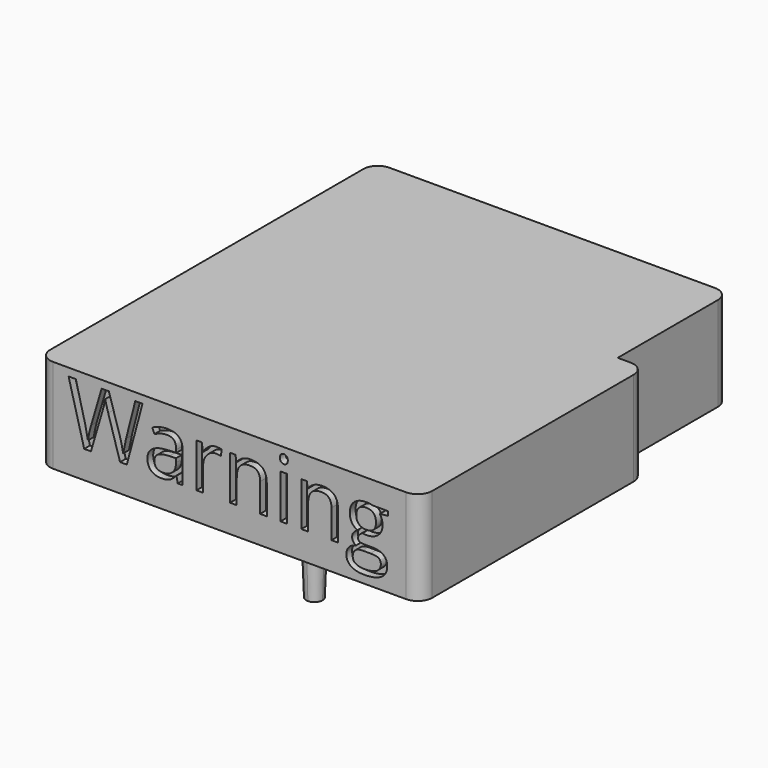
from build123d import *

# Parameters (mm, degrees)
F1_DEPTH     = 10
F2_DEPTH     = 3
F3_DEPTH     = 15
F3_TAPER     = 2
F4_TEXT_SIZE = 11.36543015
F5_DEPTH     = 1


# Not quite as in the source:
# - Text() gives the source's letters only with a copy of the font that has no kerning and outlines rounded to 1/6400 em; it was checked with that copy


with BuildPart() as f1:
    # F0 (on Top) → F1 (new body)
    with BuildSketch(Plane.XY):
        with BuildLine():
            Line((0, 34.5), (0, 0))
            Line((0, 0), (-15, 0))
            ThreePointArc((-15, 0), (-13.833273811, -0.483273811), (-13.35, -1.65))
            ThreePointArc((-13.35, -1.65), (-13.8332738152, -2.8167261931), (-15.0000000118, -3.3))
            Line((-15.0000000118, -3.3), (-1, -3.3))
            ThreePointArc((-1, -3.3), (0.4142135624, -2.7142135624), (1, -1.3))
            Line((1, -1.3), (1, 33.5))
            ThreePointArc((1, 33.5), (0.4142135624, 34.9142135624), (-1, 35.5))
            Line((-1, 35.5), (-2.81, 35.5))
            Line((-2.81, 35.5), (-2.81, 52.8))
            ThreePointArc((-2.81, 52.8), (-3.3957864376, 54.2142135624), (-4.81, 54.8))
            Line((-4.81, 54.8), (-16.51, 54.8))
            ThreePointArc((-16.51, 54.8), (-15.343273811, 54.316726189), (-14.86, 53.15))
            ThreePointArc((-14.86, 53.15), (-15.343273811, 51.983273811), (-16.51, 51.5))
            Line((-16.51, 51.5), (-3.81, 51.5))
            Line((-3.81, 51.5), (-3.81, 34.5))
            Line((-3.81, 34.5), (0, 34.5))
        make_face()
        with BuildLine():
            ThreePointArc((-15.0000000118, -3.3), (-16.65, -1.6499999941), (-15, 0))
            Line((-15, 0), (-50.8, 0))
            Line((-50.8, 0), (-50.8, 51.5))
            Line((-50.8, 51.5), (-16.51, 51.5))
            ThreePointArc((-16.51, 51.5), (-18.16, 53.15), (-16.51, 54.8))
            Line((-16.51, 54.8), (-49.8, 54.8))
            ThreePointArc((-49.8, 54.8), (-51.2142135624, 54.2142135624), (-51.8, 52.8))
            Line((-51.8, 52.8), (-51.8, -1.3))
            ThreePointArc((-51.8, -1.3), (-51.2142135624, -2.7142135624), (-49.8, -3.3))
            Line((-49.8, -3.3), (-15.0000000118, -3.3))
        make_face()
        with BuildLine():
            ThreePointArc((-16.51, 54.8), (-18.16, 53.15), (-16.51, 51.5))
            ThreePointArc((-16.51, 51.5), (-15.343273811, 51.983273811), (-14.86, 53.15))
            ThreePointArc((-14.86, 53.15), (-15.343273811, 54.316726189), (-16.51, 54.8))
        make_face()
        with BuildLine():
            ThreePointArc((-13.35, -1.65), (-13.833273811, -0.483273811), (-15, 0))
            ThreePointArc((-15, 0), (-16.65, -1.6499999941), (-15.0000000118, -3.3))
            ThreePointArc((-15.0000000118, -3.3), (-13.8332738152, -2.8167261931), (-13.35, -1.65))
        make_face()
    extrude(amount=-F1_DEPTH)

    # F0 (on Top) → F2 (join)
    with BuildSketch(Plane.XY):
        with BuildLine():
            Line((0, 34.5), (0, 0))
            Line((0, 0), (-15, 0))
            ThreePointArc((-15, 0), (-13.833273811, -0.483273811), (-13.35, -1.65))
            ThreePointArc((-13.35, -1.65), (-13.8332738152, -2.8167261931), (-15.0000000118, -3.3))
            Line((-15.0000000118, -3.3), (-1, -3.3))
            ThreePointArc((-1, -3.3), (0.4142135624, -2.7142135624), (1, -1.3))
            Line((1, -1.3), (1, 33.5))
            ThreePointArc((1, 33.5), (0.4142135624, 34.9142135624), (-1, 35.5))
            Line((-1, 35.5), (-2.81, 35.5))
            Line((-2.81, 35.5), (-2.81, 52.8))
            ThreePointArc((-2.81, 52.8), (-3.3957864376, 54.2142135624), (-4.81, 54.8))
            Line((-4.81, 54.8), (-16.51, 54.8))
            ThreePointArc((-16.51, 54.8), (-15.343273811, 54.316726189), (-14.86, 53.15))
            ThreePointArc((-14.86, 53.15), (-15.343273811, 51.983273811), (-16.51, 51.5))
            Line((-16.51, 51.5), (-3.81, 51.5))
            Line((-3.81, 51.5), (-3.81, 34.5))
            Line((-3.81, 34.5), (0, 34.5))
        make_face()
        with BuildLine():
            ThreePointArc((-15.0000000118, -3.3), (-16.65, -1.6499999941), (-15, 0))
            Line((-15, 0), (-50.8, 0))
            Line((-50.8, 0), (-50.8, 51.5))
            Line((-50.8, 51.5), (-16.51, 51.5))
            ThreePointArc((-16.51, 51.5), (-18.16, 53.15), (-16.51, 54.8))
            Line((-16.51, 54.8), (-49.8, 54.8))
            ThreePointArc((-49.8, 54.8), (-51.2142135624, 54.2142135624), (-51.8, 52.8))
            Line((-51.8, 52.8), (-51.8, -1.3))
            ThreePointArc((-51.8, -1.3), (-51.2142135624, -2.7142135624), (-49.8, -3.3))
            Line((-49.8, -3.3), (-15.0000000118, -3.3))
        make_face()
        with BuildLine():
            ThreePointArc((-13.35, -1.65), (-13.833273811, -0.483273811), (-15, 0))
            ThreePointArc((-15, 0), (-16.65, -1.6499999941), (-15.0000000118, -3.3))
            ThreePointArc((-15.0000000118, -3.3), (-13.8332738152, -2.8167261931), (-13.35, -1.65))
        make_face()
        with BuildLine():
            ThreePointArc((-16.51, 54.8), (-18.16, 53.15), (-16.51, 51.5))
            ThreePointArc((-16.51, 51.5), (-15.343273811, 51.983273811), (-14.86, 53.15))
            ThreePointArc((-14.86, 53.15), (-15.343273811, 54.316726189), (-16.51, 54.8))
        make_face()
        Polygon((-15, 0), (0, 0), (0, 34.5), (-3.81, 34.5), (-3.81, 51.5), (-16.51, 51.5), (-50.8, 51.5), (-50.8, 0), align=None)
    extrude(amount=F2_DEPTH)

    # F0 (on Top) → F3 (join)
    with BuildSketch(Plane.XY):
        with BuildLine():
            ThreePointArc((-13.35, -1.65), (-13.833273811, -0.483273811), (-15, 0))
            ThreePointArc((-15, 0), (-16.65, -1.6499999941), (-15.0000000118, -3.3))
            ThreePointArc((-15.0000000118, -3.3), (-13.8332738152, -2.8167261931), (-13.35, -1.65))
        make_face()
        with BuildLine():
            ThreePointArc((-16.51, 54.8), (-18.16, 53.15), (-16.51, 51.5))
            ThreePointArc((-16.51, 51.5), (-15.343273811, 51.983273811), (-14.86, 53.15))
            ThreePointArc((-14.86, 53.15), (-15.343273811, 54.316726189), (-16.51, 54.8))
        make_face()
    extrude(amount=-F3_DEPTH, taper=F3_TAPER)

    # F4 (on face) → F5 (cut)
    with BuildSketch(Plane.XZ.offset(3.3)):
        with Locations((-47.8, -6.183109708)):
            Text('Warning', F4_TEXT_SIZE, font='Open Sans', text_align=(TextAlign.LEFT, TextAlign.BOTTOM))
    extrude(amount=-F5_DEPTH, mode=Mode.SUBTRACT)


solid = f1.part
